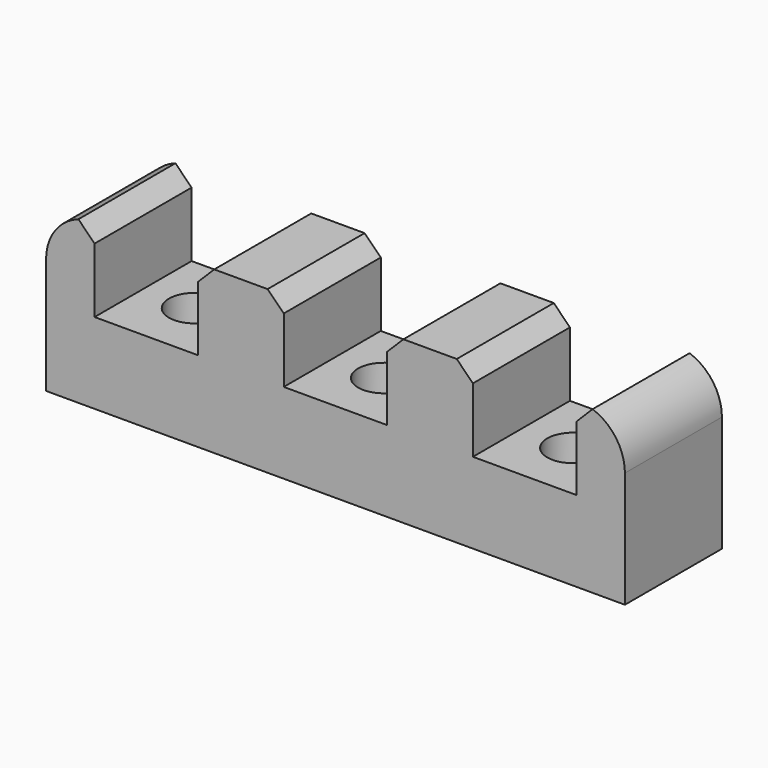
from build123d import *

# Parameters (mm, degrees)
F1_DEPTH    = 7.5
F2_SIZE     = 1
F3_T1_DEPTH = 21.6421356237
F4_R        = 1.6
F5_DEPTH    = 5.001
F6_R        = 1.6
F7_DEPTH    = 5.001
F8_R        = 1.6
F9_DEPTH    = 5.001
F10_R       = 2.85
F10_R_2     = 1.6
F11_DEPTH   = 3


# Not quite as in the source:
# - a fillet or chamfer that OpenCascade refuses, or shapes differently, is made with other operations: its cross-section is extruded or revolved along the edge and cut away or added


with BuildPart() as f1:
    # F0 (on Front) → F1 (new body)
    with BuildSketch(Plane.XZ):
        Polygon((0, 10), (0, 0), (35.8, 0), (35.8, 10), (32.8, 10), (32.8, 5), (26.4, 5), (26.4, 10), (21.1, 10), (21.1, 5), (14.7, 5), (14.7, 10), (9.4, 10), (9.4, 5), (3, 5), (3, 10), align=None)
    extrude(amount=F1_DEPTH)

    # F2
    f2_edges = [f1.edges().sort_by_distance(p)[0] for p in [
        (3, -3.75, 10),
        (9.4, -3.75, 10),
        (14.7, -3.75, 10),
        (21.1, -3.75, 10),
        (26.4, -3.75, 10),
        (32.8, -3.75, 10),
    ]]
    chamfer(f2_edges, length=F2_SIZE)

    # F3: fillet of radius 3 on 2 edges, made by hand

    # F3_s2 → F3_t1 (cut)
    with BuildSketch(Plane.XZ.offset(-7.0710678119)):
        with BuildLine():
            ThreePointArc((0, 7.1715728753), (0.5505102572, 8.9036236828), (2, 10))
            Line((2, 10), (0, 10))
            Line((0, 10), (0, 7.1715728753))
        make_face()
        with BuildLine():
            ThreePointArc((33.8, 10), (35.2494897428, 8.9036236828), (35.8, 7.1715728753))
            Line((35.8, 7.1715728753), (35.8, 10))
            Line((35.8, 10), (33.8, 10))
        make_face()
    extrude(amount=F3_T1_DEPTH, mode=Mode.SUBTRACT)

    # F4 (on face) → F5 (cut, through all)
    with BuildSketch(Plane.XY.offset(5)):
        with Locations((6.2, -3.75)):
            Circle(F4_R)
    extrude(amount=-F5_DEPTH, mode=Mode.SUBTRACT)

    # F6 (on face) → F7 (cut, through all)
    with BuildSketch(Plane.XY.offset(5)):
        with Locations((17.9, -3.75)):
            Circle(F6_R)
    extrude(amount=-F7_DEPTH, mode=Mode.SUBTRACT)

    # F8 (on face) → F9 (cut, through all)
    with BuildSketch(Plane.XY.offset(5)):
        with Locations((29.6, -3.75)):
            Circle(F8_R)
    extrude(amount=-F9_DEPTH, mode=Mode.SUBTRACT)

    # F10 (on face) → F11 (cut)
    with BuildSketch(Plane(origin=(0, 0, 0), x_dir=(1, 0, 0), z_dir=(0, 0, -1))):
        with Locations((6.2, 3.75)):
            Circle(F10_R)
        with Locations((6.2, 3.75)):
            Circle(F10_R_2, mode=Mode.SUBTRACT)
        with Locations((17.9, 3.75)):
            Circle(F10_R)
        with Locations((17.9, 3.75)):
            Circle(F10_R_2, mode=Mode.SUBTRACT)
        with Locations((29.6, 3.75)):
            Circle(F10_R)
        with Locations((29.6, 3.75)):
            Circle(F10_R_2, mode=Mode.SUBTRACT)
    extrude(amount=-F11_DEPTH, mode=Mode.SUBTRACT)


solid = f1.part
